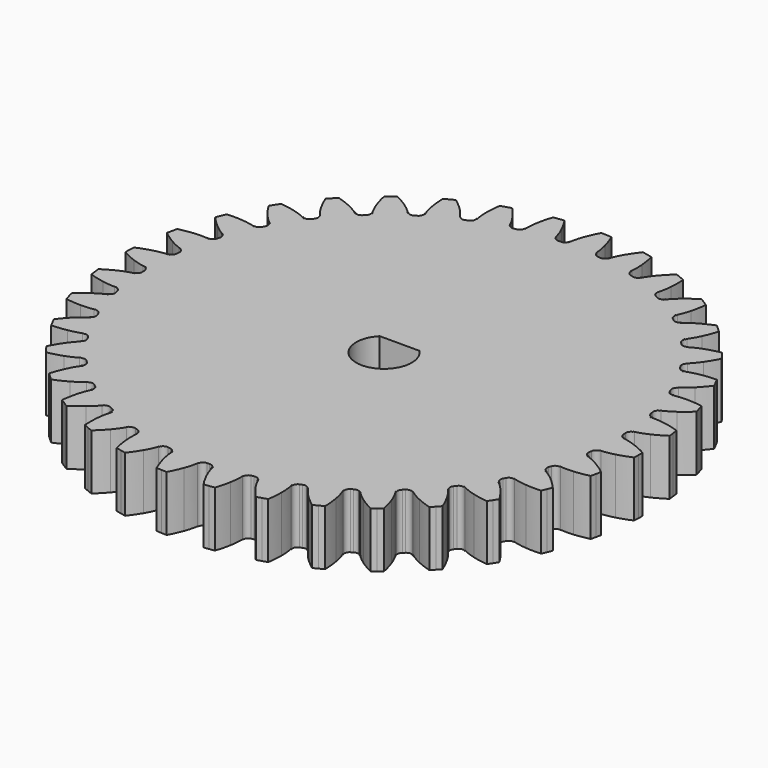
from build123d import *

# Parameters (mm, degrees)
F1_R            = 20.9375
F2_DEPTH        = 5
F4_DEPTH        = 5.001
F6_DEPTH        = 5
F6_COPIES_COUNT = 36


# Not quite as in the source:
# - a pattern or mirror of a feature is missing from the dataset's text; its kind, count and spacing are read off the source's solid


with BuildPart() as f2:
    # F1 (on Top) → F2 (new body)
    with BuildSketch(Plane.XY):
        Circle(F1_R)
    extrude(amount=F2_DEPTH)

    # F3 (on face) → F4 (cut, through all)
    with BuildSketch(Plane.XY.offset(5)):
        with BuildLine():
            Line((1.7853571071, 1.75), (-1.7853571071, 1.75))
            ThreePointArc((-1.7853571071, 1.75), (0, -2.5), (1.7853571071, 1.75))
        make_face()
    extrude(amount=-F4_DEPTH, mode=Mode.SUBTRACT)

    # F5 (on Top) → F6 (join)
    with BuildSketch(Plane.XY):
        with BuildLine():
            ThreePointArc((1.0362892257, 23.7273809056), (0.802638016, 23.736433435), (0.5689090061, 23.7431851811))
            ThreePointArc((0.5689090061, 23.7431851811), (0.2618784806, 23.1319238772), (0, 22.5))
            ThreePointArc((0, 22.5), (0.9817476875, 22.4785713843), (1.9616253755, 22.4143263536))
            ThreePointArc((1.9616253755, 22.4143263536), (1.7558372948, 23.0666754864), (1.503267663, 23.7023772296))
            ThreePointArc((1.503267663, 23.7023772296), (1.2698399875, 23.7160284703), (1.0362892257, 23.7273809056))
        make_face()
        with BuildLine():
            ThreePointArc((1.9616253755, 22.4143263536), (0.9817476875, 22.4785713843), (0, 22.5))
            ThreePointArc((0, 22.5), (-0.2082183246, 21.8298884651), (-0.3385034528, 21.1403740524))
            Line((-0.3385034528, 21.1403740524), (-0.3426345957, 21.3983740979))
            ThreePointArc((-0.3426345957, 21.3983740979), (-0.471053493, 21.0684686787), (-0.7935582856, 20.9224561536))
            ThreePointArc((-0.7935582856, 20.9224561536), (0.9135707648, 20.9175594826), (2.6146264579, 20.7736042789))
            ThreePointArc((2.6146264579, 20.7736042789), (2.3060795336, 20.9471778778), (2.2069118788, 21.2870231))
            Line((2.2069118788, 21.2870231), (2.1803031579, 21.0303656127))
            ThreePointArc((2.1803031579, 21.0303656127), (2.1106282951, 21.7286132431), (1.9616253755, 22.4143263536))
        make_face()
    f6 = extrude(amount=F6_DEPTH)

    # F6_copies: F6 ×36 about axis
    f6_copies_axis = Axis((0, 0, 0), (0, 0, 1))
    for i in range(1, F6_COPIES_COUNT):
        add(f6.rotate(f6_copies_axis, i * 360 / F6_COPIES_COUNT))


solid = f2.part
